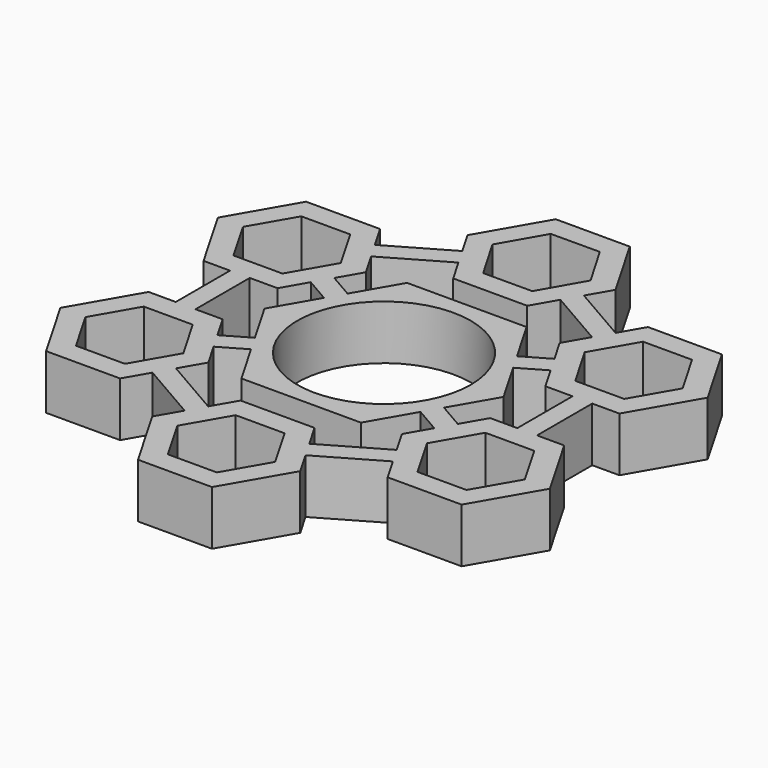
from build123d import *

# Parameters (mm, degrees)
F0_W     = 2.54
F0_H     = 8.7372876405
F0_H_2   = 8.89
F1_DEPTH = 6.9977
F2_R     = 11.176
F3_DEPTH = 6.9977


with BuildPart() as f1:
    # F0 (on Top) → F1 (new body)
    with BuildSketch(Plane.XY):
        Polygon((-11.6335226281, 5.2501477372), (-10.3635226281, 7.4498522628), (-14.0807527651, 9.595996083), (-15.3507527651, 7.3962915574), align=None)
        Polygon((-15.3507527651, 7.3962915574), (-14.0807527651, 9.595996083), (-12.3768237899, 12.5472876405), (-14.124837026, 15.5749353777), (-14.2130055479, 15.7276477372), (-15.394837026, 17.7746399033), (-17.1428502621, 20.8022876405), (-26.6749032064, 20.8022876405), (-31.4409296786, 12.5472876405), (-26.6749032064, 4.2922876405), (-23.2670452561, 4.2922876405), (-20.7270452561, 4.2922876405), (-17.1428502621, 4.2922876405), align=None)
        Polygon((-18.7559669142, 18.0082876405), (-15.6030570942, 12.5472876405), (-18.7559669142, 7.0862876405), (-25.0617865543, 7.0862876405), (-28.2146963743, 12.5472876405), (-25.0617865543, 18.0082876405), align=None, mode=Mode.SUBTRACT)
        Polygon((14.2130055479, 9.6723522628), (10.3635226281, 7.4498522628), (11.6335226281, 5.2501477372), (15.4830055479, 7.4726477372), align=None)
        Polygon((-10.3635226281, -7.4498522628), (-11.6335226281, -5.2501477372), (-15.4830055479, -7.4726477372), (-14.2130055479, -9.6723522628), align=None)
        Polygon((-14.2130055479, 15.7276477372), (-14.124837026, 15.5749353777), (-6.4258711864, 20.0199353777), (-7.6958711864, 22.2196399033), (-15.394837026, 17.7746399033), align=None)
        Polygon((12.4649923118, 12.7), (14.2130055479, 9.6723522628), (15.4830055479, 7.4726477372), (17.231018784, 4.445), (20.7270452561, 4.445), (23.2670452561, 4.445), (26.7630717283, 4.445), (31.5290982004, 12.7), (26.7630717283, 20.955), (17.231018784, 20.955), (15.4830055479, 17.9273522628), (14.2130055479, 15.7276477372), align=None)
        Polygon((25.1499550762, 7.239), (18.8441354361, 7.239), (15.691225616, 12.7), (18.8441354361, 18.161), (25.1499550762, 18.161), (28.3028648962, 12.7), align=None, mode=Mode.SUBTRACT)
        Polygon((-14.2130055479, -9.6723522628), (-15.4830055479, -7.4726477372), (-17.231018784, -4.445), (-20.7270452561, -4.445), (-23.2670452561, -4.445), (-26.7630717283, -4.445), (-31.5290982004, -12.7), (-26.7630717283, -20.955), (-17.231018784, -20.955), (-15.4830055479, -17.9273522628), (-14.2130055479, -15.7276477372), (-12.4649923118, -12.7), align=None)
        Polygon((-25.1499550762, -7.239), (-18.8441354361, -7.239), (-15.691225616, -12.7), (-18.8441354361, -18.161), (-25.1499550762, -18.161), (-28.3028648962, -12.7), align=None, mode=Mode.SUBTRACT)
        with Locations((-21.9970452561, -0.0763561798)):
            Rectangle(F0_W, F0_H)
        Polygon((-7.6958711864, 22.2196399033), (-6.4258711864, 20.0199353777), (-4.6778579503, 16.9922876405), (-1.27, 16.9922876405), (1.27, 16.9922876405), (4.854194994, 16.9922876405), (6.6462924911, 20.0962915574), (7.9162924911, 22.295996083), (9.6202214662, 25.2472876405), (4.854194994, 33.5022876405), (-4.6778579503, 33.5022876405), (-9.4438844224, 25.2472876405), align=None)
        Polygon((6.3939514928, 25.2687924658), (3.2596837324, 19.7970718096), (-3.0460992385, 19.7755669843), (-6.217614449, 25.2257828151), (-3.0833466886, 30.6975034713), (3.2224362823, 30.7190082967), align=None, mode=Mode.SUBTRACT)
        Polygon((15.4830055479, -7.4726477372), (11.6335226281, -5.2501477372), (10.3635226281, -7.4498522628), (14.2130055479, -9.6723522628), align=None)
        Polygon((6.6462924911, 20.0962915574), (14.2130055479, 15.7276477372), (15.4830055479, 17.9273522628), (7.9162924911, 22.295996083), align=None)
        Polygon((17.231018784, -4.445), (15.4830055479, -7.4726477372), (14.2130055479, -9.6723522628), (12.4649923118, -12.7), (14.2130055479, -15.7276477372), (15.4830055479, -17.9273522628), (17.231018784, -20.955), (26.7630717283, -20.955), (31.5290982004, -12.7), (26.7630717283, -4.445), (23.2670452561, -4.445), (20.7270452561, -4.445), align=None)
        Polygon((18.8441354361, -18.161), (15.691225616, -12.7), (18.8441354361, -7.239), (25.1499550762, -7.239), (28.3028648962, -12.7), (25.1499550762, -18.161), align=None, mode=Mode.SUBTRACT)
        with Locations((21.9970452561, 0)):
            Rectangle(F0_W, F0_H_2)
        Polygon((-6.5140397082, -20.1726477372), (-14.2130055479, -15.7276477372), (-15.4830055479, -17.9273522628), (-7.7840397082, -22.3723522628), align=None)
        Polygon((-4.7660264722, -17.145), (-6.5140397082, -20.1726477372), (-7.7840397082, -22.3723522628), (-9.5320529443, -25.4), (-4.7660264722, -33.655), (4.7660264722, -33.655), (9.5320529443, -25.4), (7.7840397082, -22.3723522628), (6.5140397082, -20.1726477372), (4.7660264722, -17.145), (1.27, -17.145), (-1.27, -17.145), align=None)
        Polygon((-6.3058196401, -25.4), (-3.15290982, -19.939), (3.15290982, -19.939), (6.3058196401, -25.4), (3.15290982, -30.861), (-3.15290982, -30.861), align=None, mode=Mode.SUBTRACT)
        Polygon((15.4830055479, -17.9273522628), (14.2130055479, -15.7276477372), (6.5140397082, -20.1726477372), (7.7840397082, -22.3723522628), align=None)
    extrude(amount=F1_DEPTH)

    # F2 (on Top) → F3 (join)
    with BuildSketch(Plane.XY):
        Polygon((7.6989658396, 13.335), (-7.6989658396, 13.335), (-15.3979316793, 0), (-7.6989658396, -13.335), (7.6989658396, -13.335), (15.3979316793, 0), align=None)
        Circle(F2_R, mode=Mode.SUBTRACT)
    extrude(amount=F3_DEPTH)


solid = f1.part
